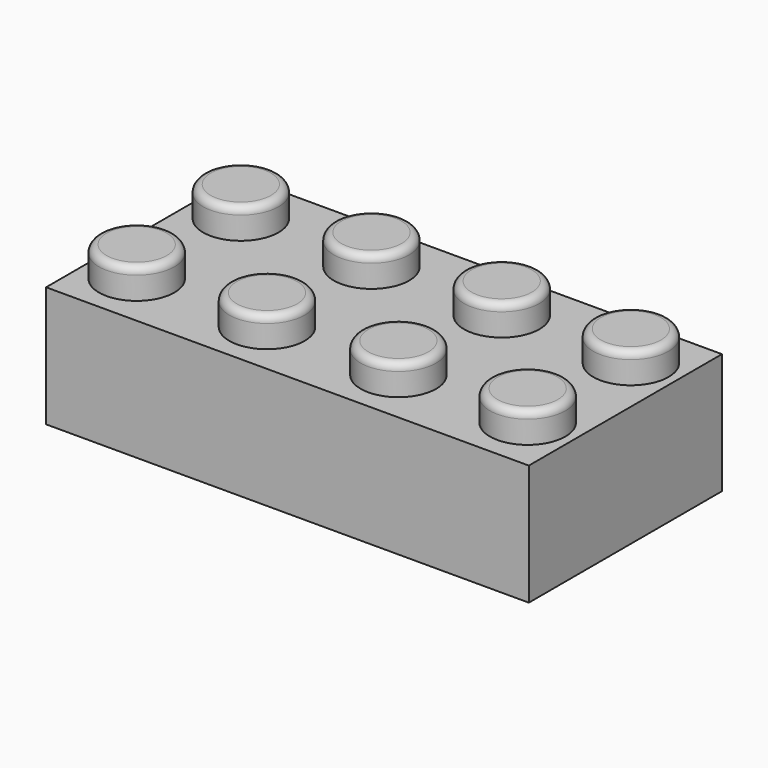
from build123d import *

# Parameters (mm, degrees)
F0_W        = 32
F0_H        = 16
F1_DEPTH    = 8
F3_R        = 2.5
F4_DEPTH    = 2
F6_R        = 0.5
F7_T        = -1.5
F5_R        = 3
F8_DEPTH    = 8
F9_T        = 1
F9_T3_DEPTH = 8.5
F9_T5_DEPTH = 31
F9_T7_DEPTH = 15


# Not quite as in the source:
# - a shell that OpenCascade refuses in one call is made with other operations: the cavity is built on its own and cut out


with BuildPart() as f1:
    # F0 (on Top) → F1 (new body)
    with BuildSketch(Plane.XY):
        Rectangle(F0_W, F0_H)
    extrude(amount=F1_DEPTH)

    # F3 (on offset) → F4 (join)
    with BuildSketch(Plane.XY.offset(8)):
        with Locations((-12.94234666, 4.3141155533)):
            Circle(F3_R)
        with Locations((-4.2926156893, 4.3285023421)):
            Circle(F3_R)
        with Locations((4.3787667528, 4.2801434174)):
            Circle(F3_R)
        with Locations((12.945256196, 4.276055377)):
            Circle(F3_R)
        with Locations((12.945256196, -4.276055377)):
            Circle(F3_R)
        with Locations((4.3787667528, -4.2801434174)):
            Circle(F3_R)
        with Locations((-4.2926156893, -4.3285023421)):
            Circle(F3_R)
        with Locations((-12.94234666, -4.3141155533)):
            Circle(F3_R)
    extrude(amount=F4_DEPTH)

    # F6
    f6_edges = [f1.edges().sort_by_distance(p)[0] for p in [
        (-15.442347, 4.314116, 10),
        (-15.442347, -4.314116, 10),
        (-6.792616, -4.328502, 10),
        (-6.792616, 4.328502, 10),
        (1.878767, 4.280143, 10),
        (1.878767, -4.280143, 10),
        (10.445256, 4.276055, 10),
        (10.445256, -4.276055, 10),
    ]]
    fillet(f6_edges, radius=F6_R)

    # F7
    f7_openings = [f1.faces().sort_by_distance(p)[0] for p in [
        (0, 0, 0),
    ]]
    offset(amount=F7_T, openings=f7_openings, kind=Kind.INTERSECTION)

    # F5 (on Top) → F8 (join)
    with BuildSketch(Plane.XY):
        with Locations((-8, 0)):
            Circle(F5_R)
        Circle(F5_R)
        with Locations((8, 0)):
            Circle(F5_R)
    extrude(amount=F8_DEPTH)

    # F9: shell of thickness 1, made by hand


with BuildPart() as f9_core1:
    # F9_t2: copy of F1
    add(f1.part)

    # the walls: a layer under each face that stays
    f9_faces = [f9_core1.faces().sort_by_distance(p)[0] for p in [
        (-15.44234666, -4.3141155533, 8.75),
        (0, 0, 8),
        (-12.94234666, -4.3141155533, 10),
        (0, -8, 4),
        (-16, 0, 4),
        (16, 0, 4),
        (0, 8, 4),
        (-6.7926156893, -4.3285023421, 8.75),
        (1.8787667528, -4.2801434174, 8.75),
        (10.445256196, -4.276055377, 8.75),
        (-15.44234666, 4.3141155533, 8.75),
        (-6.7926156893, 4.3285023421, 8.75),
        (1.8787667528, 4.2801434174, 8.75),
        (10.445256196, 4.276055377, 8.75),
        (-13.7142857143, -6.8571428571, 0),
        (0, -6.5, 3.25),
        (-14.5, 0, 3.25),
        (0, 6.5, 3.25),
        (14.5, 0, 3.25),
        (-4.2926156893, -4.3285023421, 10),
        (4.3787667528, -4.2801434174, 10),
        (12.945256196, -4.276055377, 10),
        (-12.94234666, 4.3141155533, 10),
        (-4.2926156893, 4.3285023421, 10),
        (4.3787667528, 4.2801434174, 10),
        (12.945256196, 4.276055377, 10),
        (-9.6666666667, -4.3333333333, 6.5),
        (-13.94234666, -4.3141155533, 7.5),
        (-5.2926156893, -4.3285023421, 7.5),
        (3.3787667528, -4.2801434174, 7.5),
        (11.945256196, -4.276055377, 7.5),
        (-11, 0, 3.25),
        (-3, 0, 3.25),
        (-13.94234666, 4.3141155533, 7.5),
        (-5.2926156893, 4.3285023421, 7.5),
        (5, 0, 3.25),
        (3.3787667528, 4.2801434174, 7.5),
        (11.945256196, 4.276055377, 7.5),
        (-12.94234666, -4.3141155533, 8.5),
        (-4.2926156893, -4.3285023421, 8.5),
        (4.3787667528, -4.2801434174, 8.5),
        (12.945256196, -4.276055377, 8.5),
        (-12.94234666, 4.3141155533, 8.5),
        (-4.2926156893, 4.3285023421, 8.5),
        (4.3787667528, 4.2801434174, 8.5),
        (12.945256196, 4.276055377, 8.5),
    ]]
    thicken(f9_faces, amount=-F9_T, mode=Mode.SUBTRACT)

    # F9_s4 → F9_t3 (cut)
    with BuildSketch(Plane.XY.offset(-1)):
        Polygon((-14.49, -6.49), (-14.5, -7.5), (-15.5, -7.5), (-15.5, -6.5), align=None)
        Polygon((14.49, -6.49), (14.5, -7.5), (15.5, -7.5), (15.5, -6.5), align=None)
        Polygon((-14.49, 6.49), (-15.5, 6.5), (-15.5, 7.5), (-14.5, 7.5), align=None)
        Polygon((14.49, 6.49), (14.5, 7.5), (15.5, 7.5), (15.5, 6.5), align=None)
    extrude(amount=F9_T3_DEPTH, mode=Mode.SUBTRACT)

    # F9_s6 → F9_t5 (cut)
    with BuildSketch(Plane.YZ.offset(-15.5)):
        Polygon((-6.49, 6.49), (-7.5, 6.5), (-7.5, 7.5), (-6.5, 7.5), align=None)
        Polygon((6.49, 6.49), (7.5, 6.5), (7.5, 7.5), (6.5, 7.5), align=None)
    extrude(amount=F9_T5_DEPTH, mode=Mode.SUBTRACT)

    # F9_s8 → F9_t7 (cut)
    with BuildSketch(Plane.XZ.offset(-7.5)):
        Polygon((-14.49, 6.49), (-15.5, 6.5), (-15.5, 7.5), (-14.5, 7.5), align=None)
        Polygon((14.49, 6.49), (15.5, 6.5), (15.5, 7.5), (14.5, 7.5), align=None)
    extrude(amount=F9_T7_DEPTH, mode=Mode.SUBTRACT)

    # F9_s9 → F9_t10 (revolve, cut)
    with BuildSketch(Plane.XZ.offset(4.3141155533)):
        Polygon((-10.43234666, 8.01), (-11.44234666, 8), (-11.44234666, 7), (-10.44234666, 7), align=None)
    revolve(axis=Axis((-12.94234666, -4.3141155533, 8), (0, 0, 1)), mode=Mode.SUBTRACT)

    # F9_s11 → F9_t12 (revolve, cut)
    with BuildSketch(Plane.XZ.offset(4.3285023421)):
        Polygon((-1.7826156893, 8.01), (-1.7926156893, 7), (-2.7926156893, 7), (-2.7926156893, 8), align=None)
    revolve(axis=Axis((-4.2926156893, -4.3285023421, 8), (0, 0, 1)), mode=Mode.SUBTRACT)

    # F9_s13 → F9_t14 (revolve, cut)
    with BuildSketch(Plane.XZ.offset(4.2801434174)):
        Polygon((6.8887667528, 8.01), (6.8787667528, 7), (5.8787667528, 7), (5.8787667528, 8), align=None)
    revolve(axis=Axis((4.3787667528, -4.2801434174, 8), (0, 0, 1)), mode=Mode.SUBTRACT)

    # F9_s15 → F9_t16 (revolve, cut)
    with BuildSketch(Plane.XZ.offset(4.276055377)):
        Polygon((15.455256196, 8.01), (15.445256196, 7), (14.445256196, 7), (14.445256196, 8), align=None)
    revolve(axis=Axis((12.945256196, -4.276055377, 8), (0, 0, 1)), mode=Mode.SUBTRACT)

    # F9_s17 → F9_t18 (revolve, cut)
    with BuildSketch(Plane.XZ.offset(-4.3141155533)):
        Polygon((-10.43234666, 8.01), (-10.44234666, 7), (-11.44234666, 7), (-11.44234666, 8), align=None)
    revolve(axis=Axis((-12.94234666, 4.3141155533, 8), (0, 0, 1)), mode=Mode.SUBTRACT)

    # F9_s19 → F9_t20 (revolve, cut)
    with BuildSketch(Plane.XZ.offset(-4.3285023421)):
        Polygon((-1.7826156893, 8.01), (-1.7926156893, 7), (-2.7926156893, 7), (-2.7926156893, 8), align=None)
    revolve(axis=Axis((-4.2926156893, 4.3285023421, 8), (0, 0, 1)), mode=Mode.SUBTRACT)

    # F9_s21 → F9_t22 (revolve, cut)
    with BuildSketch(Plane.XZ.offset(-4.2801434174)):
        Polygon((6.8887667528, 8.01), (6.8787667528, 7), (5.8787667528, 7), (5.8787667528, 8), align=None)
    revolve(axis=Axis((4.3787667528, 4.2801434174, 8), (0, 0, 1)), mode=Mode.SUBTRACT)

    # F9_s23 → F9_t24 (revolve, cut)
    with BuildSketch(Plane.XZ.offset(-4.276055377)):
        Polygon((15.455256196, 8.01), (15.445256196, 7), (14.445256196, 7), (14.445256196, 8), align=None)
    revolve(axis=Axis((12.945256196, 4.276055377, 8), (0, 0, 1)), mode=Mode.SUBTRACT)

    # F9_s25 → F9_t26 (revolve, cut)
    with BuildSketch(Plane.XZ):
        Polygon((-4.99, 6.49), (-5, 7.5), (-6, 7.5), (-6, 6.5), align=None)
    revolve(axis=Axis((-8, 0, 6.5), (0, 0, -1)), mode=Mode.SUBTRACT)

    # F9_s27 → F9_t28 (revolve, cut)
    with BuildSketch(Plane.XZ):
        Polygon((3.01, 6.49), (3, 7.5), (2, 7.5), (2, 6.5), align=None)
    revolve(axis=Axis((0, 0, 6.5), (0, 0, -1)), mode=Mode.SUBTRACT)

    # F9_s29 → F9_t30 (revolve, cut)
    with BuildSketch(Plane.XZ):
        Polygon((11.01, 6.49), (11, 7.5), (10, 7.5), (10, 6.5), align=None)
    revolve(axis=Axis((8, 0, 6.5), (0, 0, -1)), mode=Mode.SUBTRACT)

    # F9_s31 → F9_t32 (revolve, cut)
    with BuildSketch(Plane.XZ.offset(4.3141155533)):
        Polygon((-11.95234666, 8.49), (-10.94234666, 8.5), (-10.94234666, 9.5), (-11.94234666, 9.5), align=None)
    revolve(axis=Axis((-12.94234666, -4.3141155533, 8.5), (0, 0, -1)), mode=Mode.SUBTRACT)

    # F9_s33 → F9_t34 (revolve, cut)
    with BuildSketch(Plane.XZ.offset(4.3285023421)):
        Polygon((-3.3026156893, 8.49), (-2.2926156893, 8.5), (-2.2926156893, 9.5), (-3.2926156893, 9.5), align=None)
    revolve(axis=Axis((-4.2926156893, -4.3285023421, 8.5), (0, 0, -1)), mode=Mode.SUBTRACT)

    # F9_s35 → F9_t36 (revolve, cut)
    with BuildSketch(Plane.XZ.offset(4.2801434174)):
        Polygon((5.3687667528, 8.49), (6.3787667528, 8.5), (6.3787667528, 9.5), (5.3787667528, 9.5), align=None)
    revolve(axis=Axis((4.3787667528, -4.2801434174, 8.5), (0, 0, -1)), mode=Mode.SUBTRACT)

    # F9_s37 → F9_t38 (revolve, cut)
    with BuildSketch(Plane.XZ.offset(4.276055377)):
        Polygon((13.935256196, 8.49), (14.945256196, 8.5), (14.945256196, 9.5), (13.945256196, 9.5), align=None)
    revolve(axis=Axis((12.945256196, -4.276055377, 8.5), (0, 0, -1)), mode=Mode.SUBTRACT)

    # F9_s39 → F9_t40 (revolve, cut)
    with BuildSketch(Plane.XZ.offset(-4.3141155533)):
        Polygon((-11.95234666, 8.49), (-10.94234666, 8.5), (-10.94234666, 9.5), (-11.94234666, 9.5), align=None)
    revolve(axis=Axis((-12.94234666, 4.3141155533, 8.5), (0, 0, -1)), mode=Mode.SUBTRACT)

    # F9_s41 → F9_t42 (revolve, cut)
    with BuildSketch(Plane.XZ.offset(-4.3285023421)):
        Polygon((-3.3026156893, 8.49), (-2.2926156893, 8.5), (-2.2926156893, 9.5), (-3.2926156893, 9.5), align=None)
    revolve(axis=Axis((-4.2926156893, 4.3285023421, 8.5), (0, 0, -1)), mode=Mode.SUBTRACT)

    # F9_s43 → F9_t44 (revolve, cut)
    with BuildSketch(Plane.XZ.offset(-4.2801434174)):
        Polygon((5.3687667528, 8.49), (6.3787667528, 8.5), (6.3787667528, 9.5), (5.3787667528, 9.5), align=None)
    revolve(axis=Axis((4.3787667528, 4.2801434174, 8.5), (0, 0, -1)), mode=Mode.SUBTRACT)

    # F9_s45 → F9_t46 (revolve, cut)
    with BuildSketch(Plane.XZ.offset(-4.276055377)):
        Polygon((13.935256196, 8.49), (14.945256196, 8.5), (14.945256196, 9.5), (13.945256196, 9.5), align=None)
    revolve(axis=Axis((12.945256196, 4.276055377, 8.5), (0, 0, -1)), mode=Mode.SUBTRACT)


with BuildPart() as f1_1:
    add(f1.part)

    # what is left inside the walls is the cavity
    f9_cavity = [f9_core1.part.solids().sort_by_distance(p)[0] for p in [
        (-9.99, 0, 4.666667),
        (-1.99, 0, 4.666667),
        (6.01, 0, 4.666667),
    ]]
    add(f9_cavity, mode=Mode.SUBTRACT)


solid = f1_1.part
